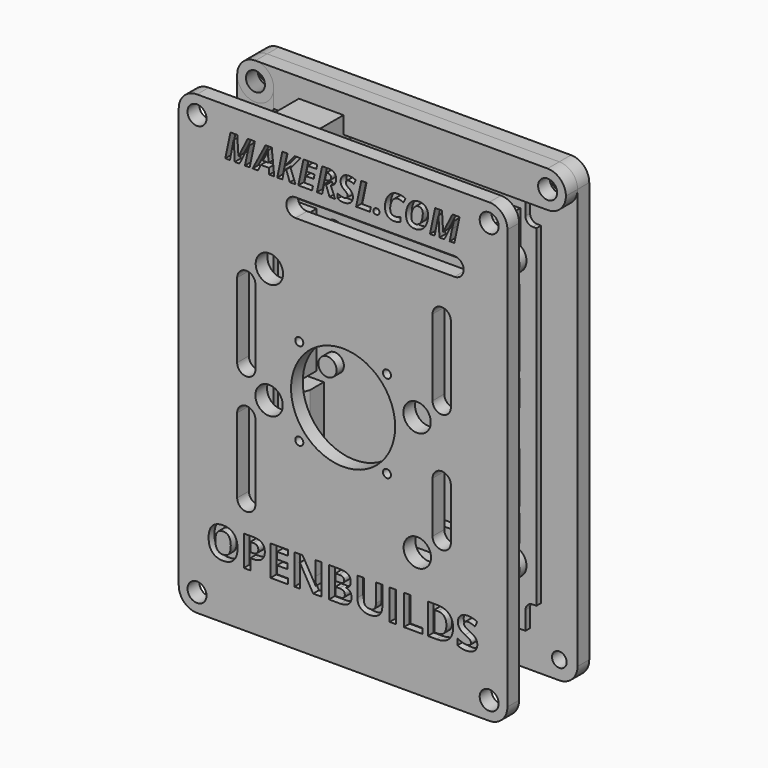
from build123d import *

# Parameters (mm, degrees)
F0_R            = 2
F0_R_2          = 1.5
F0_R_3          = 2.6
F1_DEPTH        = 4
F2_R            = 2.1
F3_DEPTH        = 4
F4_R            = 2.6
F5_DEPTH        = 4
F7_DEPTH        = 4
F8_R            = 2
F9_DEPTH        = 1.6
F10_W           = 12.2
F10_H           = 4.7
F10_H_2         = 11.8
F11_DEPTH       = 10.8
F10_W_2         = 10
F10_H_3         = 9.1
F12_DEPTH       = 12.5
F10_W_3         = 32
F10_H_4         = 7
F13_DEPTH       = 8.85
F14_SIZE2       = 4
F14_SIZE        = 1.5
F15_SIZE2       = 5
F15_SIZE        = 2
F10_W_4         = 7
F10_H_5         = 21
F16_DEPTH       = 8.8
F10_W_5         = 52.5
F10_H_6         = 9.6
F17_DEPTH       = 12.7
F10_H_7         = 14
F18_DEPTH       = 8.8
F19_SIZE2       = 4
F19_SIZE        = 1.5
F10_W_6         = 5
F10_H_8         = 7.25
F20_DEPTH       = 8.6
F21_SIZE2       = 1.5
F21_SIZE        = 4
F21_2_SIZE2     = 1.5
F21_2_SIZE      = 4
F21_3_SIZE2     = 1.5
F21_3_SIZE      = 4
F21_4_SIZE2     = 1.5
F21_4_SIZE      = 4
F21_5_SIZE2     = 1.5
F21_5_SIZE      = 4
F21_6_SIZE2     = 1.5
F21_6_SIZE      = 4
F10_R           = 2.5
F22_DEPTH       = 2.5
F23_R           = 2.6
F24_DEPTH       = 4
F26_R           = 2.6
F26_R_2         = 3.75
F27_DEPTH       = 4
F28_TEXT_SIZE   = 11.6510510219
F28_TEXT_SIZE_2 = 9.4254123618
F29_DEPTH       = 2
F30_R           = 1.1
F30_R_2         = 14.25
F31_DEPTH       = 25


# Not quite as in the source:
# - Text() gives the source's letters only with a copy of the font that has no kerning and outlines rounded to 1/6400 em; it was checked with that copy


with BuildPart() as f1:
    # F0 (on Front) → F1 (new body)
    with BuildSketch(Plane.XZ):
        with BuildLine():
            Line((-40, -62.5), (40, -62.5))
            ThreePointArc((40, -62.5), (43.5355339059, -61.0355339059), (45, -57.5))
            Line((45, -57.5), (45, 57.5))
            ThreePointArc((45, 57.5), (43.5355339059, 61.0355339059), (40, 62.5))
            Line((40, 62.5), (-40, 62.5))
            ThreePointArc((-40, 62.5), (-43.5355339059, 61.0355339059), (-45, 57.5))
            Line((-45, 57.5), (-45, -57.5))
            ThreePointArc((-45, -57.5), (-43.5355339059, -61.0355339059), (-40, -62.5))
        make_face()
        with Locations((-40, -57.5)):
            Circle(F0_R, mode=Mode.SUBTRACT)
        with Locations((-28.55, -36.75)):
            Circle(F0_R_2, mode=Mode.SUBTRACT)
        with Locations((-10, -20)):
            Circle(F0_R_3, mode=Mode.SUBTRACT)
        with Locations((40, -57.5)):
            Circle(F0_R, mode=Mode.SUBTRACT)
        with Locations((28.55, -36.75)):
            Circle(F0_R_2, mode=Mode.SUBTRACT)
        with Locations((10, -20)):
            Circle(F0_R_3, mode=Mode.SUBTRACT)
        with Locations((-10, 20)):
            Circle(F0_R_3, mode=Mode.SUBTRACT)
        with Locations((-28.55, 36.75)):
            Circle(F0_R_2, mode=Mode.SUBTRACT)
        with Locations((-40, 57.5)):
            Circle(F0_R, mode=Mode.SUBTRACT)
        with Locations((10, 20)):
            Circle(F0_R_3, mode=Mode.SUBTRACT)
        with Locations((28.55, 36.75)):
            Circle(F0_R_2, mode=Mode.SUBTRACT)
        with Locations((40, 57.5)):
            Circle(F0_R, mode=Mode.SUBTRACT)
    extrude(amount=F1_DEPTH)


with BuildPart() as f3:
    # F2 (on face) → F3 (new body)
    with BuildSketch(Plane.XZ.offset(4)):
        with BuildLine():
            ThreePointArc((-28.55, 40.5), (-32.3, 36.75), (-28.55, 33))
            Line((-28.55, 33), (28.55, 33))
            ThreePointArc((28.55, 33), (32.3, 36.75), (28.55, 40.5))
            Line((28.55, 40.5), (-28.55, 40.5))
        make_face()
        with Locations((-28.55, 36.75)):
            Circle(F2_R, mode=Mode.SUBTRACT)
        with BuildLine():
            ThreePointArc((30.65, 36.75), (28.55, 34.65), (26.45, 36.75))
            ThreePointArc((26.45, 36.75), (28.55, 38.85), (30.65, 36.75))
        make_face(mode=Mode.SUBTRACT)
    extrude(amount=F3_DEPTH)


with BuildPart() as f3b:
    # F2 (on face) → F3, piece 2 (new body)
    with BuildSketch(Plane.XZ.offset(4)):
        with BuildLine():
            ThreePointArc((-28.55, -33), (-32.3, -36.75), (-28.55, -40.5))
            Line((-28.55, -40.5), (28.55, -40.5))
            ThreePointArc((28.55, -40.5), (32.3, -36.75), (28.55, -33))
            Line((28.55, -33), (-28.55, -33))
        make_face()
        with Locations((-28.55, -36.75)):
            Circle(F2_R, mode=Mode.SUBTRACT)
        with BuildLine():
            ThreePointArc((30.65, -36.75), (28.55, -38.85), (26.45, -36.75))
            ThreePointArc((26.45, -36.75), (28.55, -34.65), (30.65, -36.75))
        make_face(mode=Mode.SUBTRACT)
    extrude(amount=F3_DEPTH)


with BuildPart() as f5:
    # F4 (on face) → F5 (new body)
    with BuildSketch(Plane.XZ.offset(4)):
        with BuildLine():
            ThreePointArc((-45, 57.5), (-43.5355339059, 53.9644660941), (-40, 52.5))
            Line((-40, 52.5), (40, 52.5))
            ThreePointArc((40, 52.5), (43.5355339059, 53.9644660941), (45, 57.5))
            ThreePointArc((45, 57.5), (43.5355339059, 61.0355339059), (40, 62.5))
            Line((40, 62.5), (-40, 62.5))
            ThreePointArc((-40, 62.5), (-43.5355339059, 61.0355339059), (-45, 57.5))
        make_face()
        with Locations((-40, 57.5)):
            Circle(F4_R, mode=Mode.SUBTRACT)
        with BuildLine():
            ThreePointArc((42.6, 57.5), (40, 54.9), (37.4, 57.5))
            ThreePointArc((37.4, 57.5), (40, 60.1), (42.6, 57.5))
        make_face(mode=Mode.SUBTRACT)
    extrude(amount=F5_DEPTH)


with BuildPart() as f7:
    # F6 (on face) → F7 (new body)
    with BuildSketch(Plane.XZ.offset(4)):
        with BuildLine():
            ThreePointArc((-40, 62.5), (-43.5355339059, 61.0355339059), (-45, 57.5))
            Line((-45, 57.5), (-45, -57.5))
            ThreePointArc((-45, -57.5), (-43.5355339059, -61.0355339059), (-40, -62.5))
            ThreePointArc((-40, -62.5), (-36.4644660941, -61.0355339059), (-35, -57.5))
            Line((-35, -57.5), (-35, 57.5))
            ThreePointArc((-35, 57.5), (-36.4644660941, 61.0355339059), (-40, 62.5))
        make_face()
        with BuildLine():
            ThreePointArc((-40, -54.9), (-38.1615223689, -55.6615223689), (-37.4, -57.5))
            ThreePointArc((-37.4, -57.5), (-41.8384776311, -59.3384776311), (-40, -54.9))
        make_face(mode=Mode.SUBTRACT)
        with BuildLine():
            ThreePointArc((-37.4, 57.5), (-38.1615223689, 55.6615223689), (-40, 54.9))
            ThreePointArc((-40, 54.9), (-41.8384776311, 59.3384776311), (-37.4, 57.5))
        make_face(mode=Mode.SUBTRACT)
    extrude(amount=F7_DEPTH)


with BuildPart() as f9:
    # F8 (on face) → F9 (new body)
    with BuildSketch(Plane.XZ.offset(4)):
        with BuildLine():
            Line((-32, -52.5), (32, -52.5))
            Line((32, -52.5), (32, -47.5))
            ThreePointArc((32, -47.5), (32.5857864376, -46.0857864376), (34, -45.5))
            Line((34, -45.5), (35, -45.5))
            Line((35, -45.5), (35, 45.5))
            Line((35, 45.5), (34, 45.5))
            ThreePointArc((34, 45.5), (32.5857864376, 46.0857864376), (32, 47.5))
            Line((32, 47.5), (32, 52.5))
            Line((32, 52.5), (-32, 52.5))
            Line((-32, 52.5), (-32, 47.5))
            ThreePointArc((-32, 47.5), (-32.5857864376, 46.0857864376), (-34, 45.5))
            Line((-34, 45.5), (-35, 45.5))
            Line((-35, 45.5), (-35, -45.5))
            Line((-35, -45.5), (-34, -45.5))
            ThreePointArc((-34, -45.5), (-32.5857864376, -46.0857864376), (-32, -47.5))
            Line((-32, -47.5), (-32, -52.5))
        make_face()
        with Locations((-28.55, -36.75)):
            Circle(F8_R, mode=Mode.SUBTRACT)
        with Locations((28.55, -36.75)):
            Circle(F8_R, mode=Mode.SUBTRACT)
        with Locations((-28.55, 36.75)):
            Circle(F8_R, mode=Mode.SUBTRACT)
        with Locations((28.55, 36.75)):
            Circle(F8_R, mode=Mode.SUBTRACT)
    extrude(amount=F9_DEPTH)


with BuildPart() as f11:
    # F10 (on face) → F11 (new body)
    with BuildSketch(Plane.XZ.offset(5.6)):
        with Locations((-22, 54.85)):
            Rectangle(F10_W, F10_H)
        with Locations((-22, 46.6)):
            Rectangle(F10_W, F10_H_2)
    extrude(amount=F11_DEPTH)


with BuildPart() as f12:
    # F10 (on face) → F12 (new body)
    with BuildSketch(Plane.XZ.offset(5.6)):
        with Locations((25.6, 44.35)):
            Rectangle(F10_W_2, F10_H_3)
    extrude(amount=F12_DEPTH)

    # F15
    f15_edges = [f12.edges().sort_by_distance(p)[0] for p in [
        (25.6, -18.1, 48.9),
    ]]
    f15_side = f12.faces().sort_by_distance((25.6, -18.1, 44.35))[0]
    chamfer(f15_edges, length=F15_SIZE, length2=F15_SIZE2, reference=f15_side)


with BuildPart() as f13:
    # F10 (on face) → F13 (new body)
    with BuildSketch(Plane.XZ.offset(5.6)):
        with Locations((2.9, 44.1)):
            Rectangle(F10_W_3, F10_H_4)
    extrude(amount=F13_DEPTH)

    # F14
    f14_edges = [f13.edges().sort_by_distance(p)[0] for p in [
        (2.9, -14.45, 47.6),
        (2.9, -14.45, 40.6),
    ]]
    f14_side = f13.faces().sort_by_distance((2.9, -14.45, 44.1))[0]
    chamfer(f14_edges, length=F14_SIZE, length2=F14_SIZE2, reference=f14_side)


with BuildPart() as f16:
    # F10 (on face) → F16 (new body)
    with BuildSketch(Plane.XZ.offset(5.6)):
        with Locations((26.85, 20)):
            Rectangle(F10_W_4, F10_H_5)
    extrude(amount=F16_DEPTH)

    # F21#3
    f21_3_edges = [f16.edges().sort_by_distance(p)[0] for p in [
        (23.35, -14.4, 20),
    ]]
    f21_3_side = f16.faces().sort_by_distance((23.35, -10, 20))[0]
    chamfer(f21_3_edges, length=F21_3_SIZE, length2=F21_3_SIZE2, reference=f21_3_side)

    # F21#4
    f21_4_edges = [f16.edges().sort_by_distance(p)[0] for p in [
        (30.35, -14.4, 20),
    ]]
    f21_4_side = f16.faces().sort_by_distance((30.35, -10, 20))[0]
    chamfer(f21_4_edges, length=F21_4_SIZE, length2=F21_4_SIZE2, reference=f21_4_side)


with BuildPart() as f16b:
    # F10 (on face) → F16, piece 2 (new body)
    with BuildSketch(Plane.XZ.offset(5.6)):
        with Locations((-26.7, 11.3)):
            Rectangle(F10_W_4, F10_H_5)
    extrude(amount=F16_DEPTH)

    # F21
    f21_edges = [f16b.edges().sort_by_distance(p)[0] for p in [
        (-30.2, -14.4, 11.3),
    ]]
    f21_side = f16b.faces().sort_by_distance((-30.2, -10, 11.3))[0]
    chamfer(f21_edges, length=F21_SIZE, length2=F21_SIZE2, reference=f21_side)

    # F21#2
    f21_2_edges = [f16b.edges().sort_by_distance(p)[0] for p in [
        (-23.2, -14.4, 11.3),
    ]]
    f21_2_side = f16b.faces().sort_by_distance((-23.2, -10, 11.3))[0]
    chamfer(f21_2_edges, length=F21_2_SIZE, length2=F21_2_SIZE2, reference=f21_2_side)


with BuildPart() as f16c:
    # F10 (on face) → F16, piece 3 (new body)
    with BuildSketch(Plane.XZ.offset(5.6)):
        with Locations((-26.7, -21)):
            Rectangle(F10_W_4, F10_H_5)
    extrude(amount=F16_DEPTH)

    # F21#5
    f21_5_edges = [f16c.edges().sort_by_distance(p)[0] for p in [
        (-30.2, -14.4, -21),
    ]]
    f21_5_side = f16c.faces().sort_by_distance((-30.2, -10, -21))[0]
    chamfer(f21_5_edges, length=F21_5_SIZE, length2=F21_5_SIZE2, reference=f21_5_side)

    # F21#6
    f21_6_edges = [f16c.edges().sort_by_distance(p)[0] for p in [
        (-23.2, -14.4, -21),
    ]]
    f21_6_side = f16c.faces().sort_by_distance((-23.2, -10, -21))[0]
    chamfer(f21_6_edges, length=F21_6_SIZE, length2=F21_6_SIZE2, reference=f21_6_side)


with BuildPart() as f17:
    # F10 (on face) → F17 (new body)
    with BuildSketch(Plane.XZ.offset(5.6)):
        with Locations((0, -46.3)):
            Rectangle(F10_W_5, F10_H_6)
    extrude(amount=F17_DEPTH)


with BuildPart() as f18:
    # F10 (on face) → F18 (new body)
    with BuildSketch(Plane.XZ.offset(5.6)):
        with Locations((26.85, -16.1)):
            Rectangle(F10_W_4, F10_H_7)
    extrude(amount=F18_DEPTH)

    # F19
    f19_edges = [f18.edges().sort_by_distance(p)[0] for p in [
        (30.35, -14.4, -16.1),
        (23.35, -14.4, -16.1),
    ]]
    f19_side = f18.faces().sort_by_distance((26.85, -14.4, -16.1))[0]
    chamfer(f19_edges, length=F19_SIZE, length2=F19_SIZE2, reference=f19_side)


with BuildPart() as f20:
    # F10 (on face) → F20 (new body)
    with BuildSketch(Plane.XZ.offset(5.6)):
        with Locations((-27.7, 27.025)):
            Rectangle(F10_W_6, F10_H_8)
    extrude(amount=F20_DEPTH)


with BuildPart() as f20b:
    # F10 (on face) → F20, piece 2 (new body)
    with BuildSketch(Plane.XZ.offset(5.6)):
        with Locations((-27.7, -4.825)):
            Rectangle(F10_W_6, F10_H_8)
    extrude(amount=F20_DEPTH)


with BuildPart() as f20c:
    # F10 (on face) → F20, piece 3 (new body)
    with BuildSketch(Plane.XZ.offset(5.6)):
        with Locations((27.85, 4.275)):
            Rectangle(F10_W_6, F10_H_8)
    extrude(amount=F20_DEPTH)


with BuildPart() as f20d:
    # F10 (on face) → F20, piece 4 (new body)
    with BuildSketch(Plane.XZ.offset(5.6)):
        with Locations((27.85, -28.325)):
            Rectangle(F10_W_6, F10_H_8)
    extrude(amount=F20_DEPTH)


with BuildPart() as f22:
    # F10 (on face) → F22 (new body)
    with BuildSketch(Plane.XZ.offset(5.6)):
        with Locations((-20.2, 27.025)):
            Circle(F10_R)
    extrude(amount=F22_DEPTH)


with BuildPart() as f22b:
    # F10 (on face) → F22, piece 2 (new body)
    with BuildSketch(Plane.XZ.offset(5.6)):
        with Locations((20.35, 4.275)):
            Circle(F10_R)
    extrude(amount=F22_DEPTH)


with BuildPart() as f22c:
    # F10 (on face) → F22, piece 3 (new body)
    with BuildSketch(Plane.XZ.offset(5.6)):
        with Locations((-20.2, -4.825)):
            Circle(F10_R)
    extrude(amount=F22_DEPTH)


with BuildPart() as f22d:
    # F10 (on face) → F22, piece 4 (new body)
    with BuildSketch(Plane.XZ.offset(5.6)):
        with Locations((20.35, -28.325)):
            Circle(F10_R)
    extrude(amount=F22_DEPTH)


with BuildPart() as f24:
    # F23 (on face) → F24 (new body)
    with BuildSketch(Plane.XZ.offset(4)):
        with BuildLine():
            ThreePointArc((-45, 57.5), (-40, 52.5), (-35, 57.5))
            ThreePointArc((-35, 57.5), (-36.4644660941, 61.0355339059), (-40, 62.5))
            ThreePointArc((-40, 62.5), (-43.5355339059, 61.0355339059), (-45, 57.5))
        make_face()
        with Locations((-40, 57.5)):
            Circle(F23_R, mode=Mode.SUBTRACT)
    extrude(amount=F24_DEPTH)


with BuildPart() as f27:
    # F26 (on offset) → F27 (new body)
    with BuildSketch(Plane.XZ.offset(24)):
        with BuildLine():
            Line((-40, -62.5), (40, -62.5))
            ThreePointArc((40, -62.5), (43.5355339059, -61.0355339059), (45, -57.5))
            Line((45, -57.5), (45, 57.5))
            ThreePointArc((45, 57.5), (43.5355339059, 61.0355339059), (40, 62.5))
            Line((40, 62.5), (-40, 62.5))
            ThreePointArc((-40, 62.5), (-43.5355339059, 61.0355339059), (-45, 57.5))
            Line((-45, 57.5), (-45, -57.5))
            ThreePointArc((-45, -57.5), (-43.5355339059, -61.0355339059), (-40, -62.5))
        make_face()
        with Locations((-40, -57.5)):
            Circle(F26_R, mode=Mode.SUBTRACT)
        with BuildLine():
            Line((-29, -31.1996527016), (-29, -10.7058370486))
            ThreePointArc((-29, -10.7058370486), (-26.5, -8.2058370486), (-24, -10.7058370486))
            Line((-24, -10.7058370486), (-24, -31.1996527016))
            ThreePointArc((-24, -31.1996527016), (-26.5, -33.6996527016), (-29, -31.1996527016))
        make_face(mode=Mode.SUBTRACT)
        with Locations((-20.2726311982, -4.8327515833)):
            Circle(F26_R_2, mode=Mode.SUBTRACT)
        with Locations((40, -57.5)):
            Circle(F26_R, mode=Mode.SUBTRACT)
        with Locations((20.3233715147, -28.3149443567)):
            Circle(F26_R_2, mode=Mode.SUBTRACT)
        with BuildLine():
            Line((24.5, -23.0461992323), (24.5, -9.053110145))
            ThreePointArc((24.5, -9.053110145), (27, -6.553110145), (29.5, -9.053110145))
            Line((29.5, -9.053110145), (29.5, -23.0461992323))
            ThreePointArc((29.5, -23.0461992323), (27, -25.5461992323), (24.5, -23.0461992323))
        make_face(mode=Mode.SUBTRACT)
        with BuildLine():
            Line((-29, 1.4001640957), (-29, 21.8920949847))
            ThreePointArc((-29, 21.8920949847), (-26.5, 24.3920949847), (-24, 21.8920949847))
            Line((-24, 21.8920949847), (-24, 1.4001640957))
            ThreePointArc((-24, 1.4001640957), (-26.5, -1.0998359043), (-29, 1.4001640957))
        make_face(mode=Mode.SUBTRACT)
        with Locations((-20.1802030206, 26.8780589104)):
            Circle(F26_R_2, mode=Mode.SUBTRACT)
        with Locations((-40, 57.5)):
            Circle(F26_R, mode=Mode.SUBTRACT)
        with Locations((20.2499870211, 4.2485971935)):
            Circle(F26_R_2, mode=Mode.SUBTRACT)
        with BuildLine():
            Line((24.5, 9.6064964309), (24.5, 30.5194072425))
            ThreePointArc((24.5, 30.5194072425), (27, 33.0194072425), (29.5, 30.5194072425))
            Line((29.5, 30.5194072425), (29.5, 9.6064964309))
            ThreePointArc((29.5, 9.6064964309), (27, 7.1064964309), (24.5, 9.6064964309))
        make_face(mode=Mode.SUBTRACT)
        with BuildLine():
            Line((30.5076725781, 41.4601838589), (-13.05074431, 41.4601838589))
            ThreePointArc((-13.05074431, 41.4601838589), (-15.55074431, 43.9601838589), (-13.05074431, 46.4601838589))
            Line((-13.05074431, 46.4601838589), (30.5076725781, 46.4601838589))
            ThreePointArc((30.5076725781, 46.4601838589), (33.0076725781, 43.9601838589), (30.5076725781, 41.4601838589))
        make_face(mode=Mode.SUBTRACT)
        with Locations((40, 57.5)):
            Circle(F26_R, mode=Mode.SUBTRACT)
    extrude(amount=F27_DEPTH)

    # F28 (on face) → F29 (cut)
    with BuildSketch(Plane.XZ.offset(28)):
        with Locations((-37.5, -47.5)):
            Text('OPENBUILDS', F28_TEXT_SIZE, font='Open Sans', font_style=FontStyle.BOLD, text_align=(TextAlign.LEFT, TextAlign.BOTTOM))
        with Locations((-32.5, 49.5820950604)):
            Text('MAKERSL.COM', F28_TEXT_SIZE_2, font='Open Sans', font_style=FontStyle.BOLDITALIC, text_align=(TextAlign.LEFT, TextAlign.BOTTOM))
    extrude(amount=-F29_DEPTH, mode=Mode.SUBTRACT)

    # F30 (on face) → F31 (cut)
    with BuildSketch(Plane.XZ.offset(28)):
        with Locations((-12, 12)):
            Circle(F30_R)
        with Locations((-12, -12)):
            Circle(F30_R)
        with Locations((12, 12)):
            Circle(F30_R)
        with Locations((12, -12)):
            Circle(F30_R)
        Circle(F30_R_2)
    extrude(amount=-F31_DEPTH, mode=Mode.SUBTRACT)


solid = Compound([f1.part, f3.part, f3b.part, f5.part, f7.part, f9.part, f11.part, f12.part, f13.part, f16.part, f16b.part, f16c.part, f17.part, f18.part, f20.part, f20b.part, f20c.part, f20d.part, f22.part, f22b.part, f22c.part, f22d.part, f24.part, f27.part])
